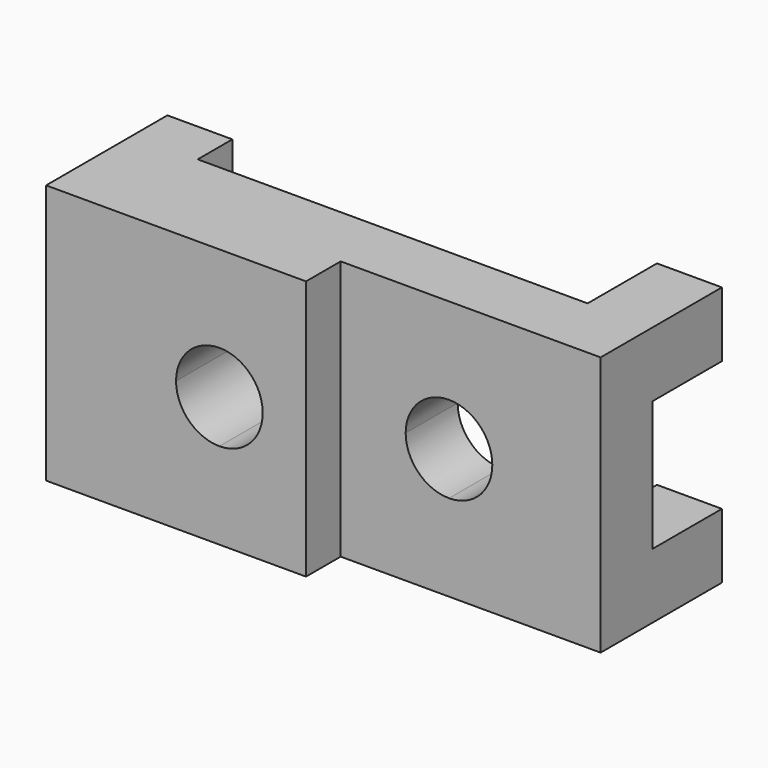
from build123d import *

# Parameters (mm, degrees)
F1_DEPTH = 30
F0_W     = 15
F0_H     = 20
F2_DEPTH = 15
F5_DEPTH = 25.001


with BuildPart() as f1:
    # F0 (on Top) → F1 (new body)
    with BuildSketch(Plane.XY):
        Polygon((-39.3988706533, 18.9813024559), (-54.3988706533, 18.9813024559), (-54.3988706533, -16.0186975441), (5.6011293467, -16.0186975441), (5.6011293467, -6.0186975441), (65.6011293467, -6.0186975441), (65.6011293467, 8.9813024559), (50.6011293467, 8.9813024559), (-39.3988706533, 8.9813024559), align=None)
    extrude(amount=F1_DEPTH)

    # F0 (on Top) → F2 (join)
    with BuildSketch(Plane.XY):
        Polygon((-39.3988706533, 18.9813024559), (-54.3988706533, 18.9813024559), (-54.3988706533, -16.0186975441), (5.6011293467, -16.0186975441), (5.6011293467, -6.0186975441), (65.6011293467, -6.0186975441), (65.6011293467, 8.9813024559), (50.6011293467, 8.9813024559), (-39.3988706533, 8.9813024559), align=None)
        with Locations((58.1011293467, 18.9813024559)):
            Rectangle(F0_W, F0_H)
    extrude(amount=F2_DEPTH)

    # F3: F1 across face


with BuildPart() as f1_1:
    add(f1.part)
    add(f1.part.mirror(Plane(origin=(-4.5459294768, -0.7245798971, 30), x_dir=(1, 0, 0), z_dir=(0, 0, 1))))

    # F4 (on face) → F5 (cut, through all)
    with BuildSketch(Plane(origin=(0, 8.9813024559, 0), x_dir=(-1, 0, 0), z_dir=(0, 1, 0))):
        with BuildLine():
            Line((-30.6011293467, 20), (-30.6011293467, 30))
            Line((-30.6011293467, 30), (-40.6011293467, 30))
            ThreePointArc((-40.6011293467, 30), (-37.6721971586, 22.9289321881), (-30.6011293467, 20))
        make_face()
        with BuildLine():
            Line((-20.6011293467, 30), (-30.6011293467, 30))
            Line((-30.6011293467, 30), (-30.6011293467, 20))
            ThreePointArc((-30.6011293467, 20), (-23.5300615349, 22.9289321881), (-20.6011293467, 30))
        make_face()
        with BuildLine():
            ThreePointArc((-20.6011293467, 30), (-23.5300615349, 37.0710678119), (-30.6011293467, 40))
            Line((-30.6011293467, 40), (-30.6011293467, 30))
            Line((-30.6011293467, 30), (-20.6011293467, 30))
        make_face()
        with BuildLine():
            Line((-30.6011293467, 30), (-30.6011293467, 40))
            ThreePointArc((-30.6011293467, 40), (-37.6721971586, 37.0710678119), (-40.6011293467, 30))
            Line((-40.6011293467, 30), (-30.6011293467, 30))
        make_face()
        with BuildLine():
            Line((24.3988706533, 30), (14.3988706533, 30))
            Line((14.3988706533, 30), (14.3988706533, 20))
            ThreePointArc((14.3988706533, 20), (21.4699384651, 22.9289321881), (24.3988706533, 30))
        make_face()
        with BuildLine():
            Line((14.3988706533, 30), (4.3988706533, 30))
            ThreePointArc((4.3988706533, 30), (7.3278028414, 22.9289321881), (14.3988706533, 20))
            Line((14.3988706533, 20), (14.3988706533, 30))
        make_face()
        with BuildLine():
            Line((14.3988706533, 30), (14.3988706533, 40))
            ThreePointArc((14.3988706533, 40), (7.3278028414, 37.0710678119), (4.3988706533, 30))
            Line((4.3988706533, 30), (14.3988706533, 30))
        make_face()
        with BuildLine():
            ThreePointArc((24.3988706533, 30), (21.4699384651, 37.0710678119), (14.3988706533, 40))
            Line((14.3988706533, 40), (14.3988706533, 30))
            Line((14.3988706533, 30), (24.3988706533, 30))
        make_face()
    extrude(amount=-F5_DEPTH, mode=Mode.SUBTRACT)


solid = f1_1.part
